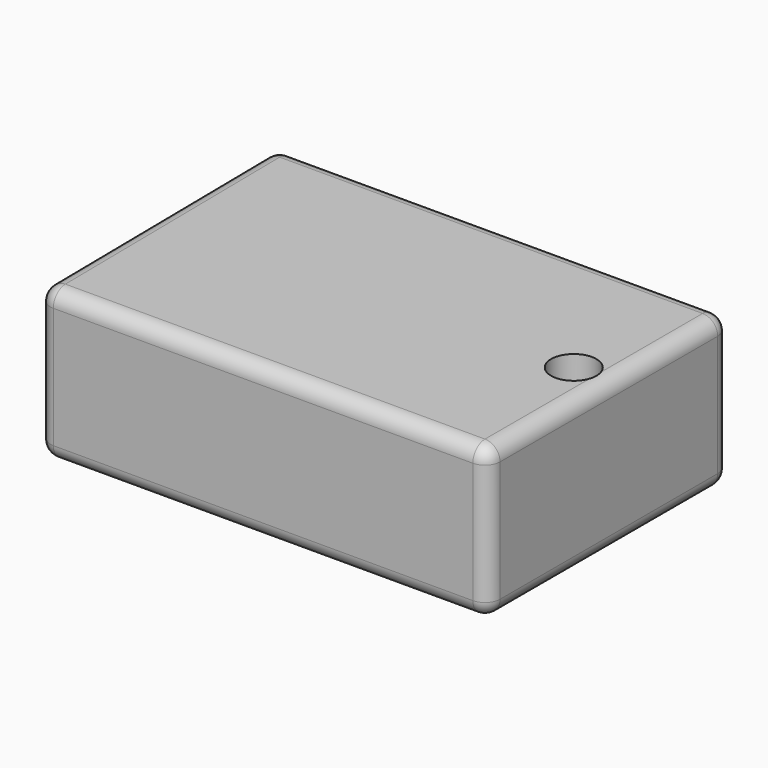
from build123d import *

# Parameters (mm, degrees)
F0_R         = 15
F1_DEPTH     = 100
F2_T1_DEPTH  = 180
F2_T3_DEPTH  = 277.5790250274
F2_T5_DEPTH  = 80
F2_T7_DEPTH  = 279.8718117474
F2_T9_DEPTH  = 180.014601827
F2_S13_W     = 10
F2_S13_H     = 10
F2_T14_DEPTH = 10
F2_S19_W     = 10
F2_S19_H     = 10
F2_T20_DEPTH = 10
F2_T26_DEPTH = 10
F2_S31_W     = 10
F2_S31_H     = 10
F2_T32_DEPTH = 10
F2_T38_DEPTH = 10
F2_S43_W     = 10
F2_S43_H     = 10
F2_T44_DEPTH = 10
F2_T50_DEPTH = 10
F2_T56_DEPTH = 10


# Not quite as in the source:
# - a fillet or chamfer that OpenCascade refuses, or shapes differently, is made with other operations: its cross-section is extruded or revolved along the edge and cut away or added


with BuildPart() as f1:
    # F0 (on Top) → F1 (new body)
    with BuildSketch(Plane.XY):
        Polygon((148.6140583592, 151.6970589757), (-151.3859416408, 151.6970589757), (-148.8384008408, -48.3029410243), (148.6140583592, -48.3029410243), align=None)
        with Locations((124.343521893, 52.9859960079)):
            Circle(F0_R, mode=Mode.SUBTRACT)
    extrude(amount=F1_DEPTH)

    # F2: fillet of radius 10 on 12 edges, made by hand

    # F2_s2 → F2_t1 (cut)
    with BuildSketch(Plane.XZ.offset(-141.6970589757)):
        with BuildLine():
            ThreePointArc((148.6140583592, 90), (145.6851261711, 97.0710678119), (138.6140583592, 100))
            Line((138.6140583592, 100), (148.6140583592, 100))
            Line((148.6140583592, 100), (148.6140583592, 90))
        make_face()
        with BuildLine():
            ThreePointArc((148.6140583592, 10), (145.6851261711, 2.9289321881), (138.6140583592, 0))
            Line((138.6140583592, 0), (148.6140583592, 0))
            Line((148.6140583592, 0), (148.6140583592, 10))
        make_face()
    extrude(amount=F2_T1_DEPTH, mode=Mode.SUBTRACT)

    # F2_s4 → F2_t3 (cut)
    with BuildSketch(Plane.YZ.offset(-138.9649666681)):
        with BuildLine():
            ThreePointArc((-48.3029410243, 90), (-45.3740088362, 97.0710678119), (-38.3029410243, 100))
            Line((-38.3029410243, 100), (-48.3029410243, 100))
            Line((-48.3029410243, 100), (-48.3029410243, 90))
        make_face()
        with BuildLine():
            ThreePointArc((-48.3029410243, 10), (-45.3740088362, 2.9289321881), (-38.3029410243, 0))
            Line((-38.3029410243, 0), (-48.3029410243, 0))
            Line((-48.3029410243, 0), (-48.3029410243, 10))
        make_face()
    extrude(amount=F2_T3_DEPTH, mode=Mode.SUBTRACT)

    # F2_s6 → F2_t5 (cut)
    with BuildSketch(Plane.XY.offset(10)):
        with BuildLine():
            ThreePointArc((138.6140583592, -48.3029410243), (145.6851261711, -45.3740088362), (148.6140583592, -38.3029410243))
            Line((148.6140583592, -38.3029410243), (148.6140583592, -48.3029410243))
            Line((148.6140583592, -48.3029410243), (138.6140583592, -48.3029410243))
        make_face()
        with BuildLine():
            ThreePointArc((148.6140583592, 141.6970589757), (145.6851261711, 148.7681267876), (138.6140583592, 151.6970589757))
            Line((138.6140583592, 151.6970589757), (148.6140583592, 151.6970589757))
            Line((148.6140583592, 151.6970589757), (148.6140583592, 141.6970589757))
        make_face()
        with BuildLine():
            ThreePointArc((-138.9649666681, -48.3029410243), (-145.9908592421, -45.4188972875), (-148.9641555213, -38.4303077322))
            Line((-148.9641555213, -38.4303077322), (-148.8384008408, -48.3029410243))
            Line((-148.8384008408, -48.3029410243), (-138.9649666681, -48.3029410243))
        make_face()
        with BuildLine():
            ThreePointArc((-141.2577533882, 151.6970589757), (-148.3737096513, 148.7229515496), (-151.2569422414, 141.5696922678))
            Line((-151.2569422414, 141.5696922678), (-151.3859416408, 151.6970589757))
            Line((-151.3859416408, 151.6970589757), (-141.2577533882, 151.6970589757))
        make_face()
    extrude(amount=F2_T5_DEPTH, mode=Mode.SUBTRACT)

    # F2_s8 → F2_t7 (cut)
    with BuildSketch(Plane.YZ.offset(-141.2577533882)):
        with BuildLine():
            ThreePointArc((151.6970589757, 10), (148.7681267876, 2.9289321881), (141.6970589757, 0))
            Line((141.6970589757, 0), (151.6970589757, 0))
            Line((151.6970589757, 0), (151.6970589757, 10))
        make_face()
        with BuildLine():
            ThreePointArc((151.6970589757, 90), (148.7681267876, 97.0710678119), (141.6970589757, 100))
            Line((141.6970589757, 100), (151.6970589757, 100))
            Line((151.6970589757, 100), (151.6970589757, 90))
        make_face()
    extrude(amount=F2_T7_DEPTH, mode=Mode.SUBTRACT)

    # F2_s10 → F2_t9 (cut)
    with BuildSketch(Plane(origin=(-1.8275176256, 143.4730800475, 0), x_dir=(0, 0, 1), z_dir=(0.0127366708, -0.9999188853, 0))):
        with BuildLine():
            ThreePointArc((10, 149.4415465191), (2.9289321881, 146.512614331), (0, 139.4415465191))
            Line((0, 139.4415465191), (0, 149.4415465191))
            Line((0, 149.4415465191), (10, 149.4415465191))
        make_face()
        with BuildLine():
            ThreePointArc((90, 149.4415465191), (97.0710678119, 146.512614331), (100, 139.4415465191))
            Line((100, 139.4415465191), (100, 149.4415465191))
            Line((100, 149.4415465191), (90, 149.4415465191))
        make_face()
    extrude(amount=F2_T9_DEPTH, mode=Mode.SUBTRACT)


with BuildPart() as f2_tool12:
    # F2_s13 → F2_t14 (new body)
    with BuildSketch(Plane.XZ.offset(38.3029410243)):
        with Locations((143.6140583592, 95)):
            Rectangle(F2_S13_W, F2_S13_H)
    extrude(amount=F2_T14_DEPTH)

    # F2_s15 → F2_t16 (revolve, cut)
    with BuildSketch(Plane(origin=(138.6140583592, -38.3029410243, 90), x_dir=(-0.7071067812, 0, -0.7071067812), z_dir=(-0.7071067812, 0, 0.7071067812))):
        with BuildLine():
            ThreePointArc((0, -10), (10, 0), (0, 10))
            Line((0, 10), (0, -10))
        make_face()
    revolve(axis=Axis((138.6140583592, -38.3029410243, 90), (0, -1, 0)), mode=Mode.SUBTRACT)


with BuildPart() as f1_1:
    add(f1.part)

    # F2_t11: cut F2_tool12
    add(f2_tool12.part, mode=Mode.SUBTRACT)


with BuildPart() as f2_tool18:
    # F2_s19 → F2_t20 (new body)
    with BuildSketch(Plane.YZ.offset(138.6140583592)):
        with Locations((146.6970589757, 95)):
            Rectangle(F2_S19_W, F2_S19_H)
    extrude(amount=F2_T20_DEPTH)

    # F2_s21 → F2_t22 (revolve, cut)
    with BuildSketch(Plane(origin=(138.6140583592, 141.6970589757, 90), x_dir=(0, -0.7071067812, -0.7071067812), z_dir=(0, -0.7071067812, 0.7071067812))):
        with BuildLine():
            ThreePointArc((0, -10), (10, 0), (0, 10))
            Line((0, 10), (0, -10))
        make_face()
    revolve(axis=Axis((138.6140583592, 141.6970589757, 90), (1, 0, 0)), mode=Mode.SUBTRACT)


with BuildPart() as f1_2:
    add(f1_1.part)

    # F2_t17: cut F2_tool18
    add(f2_tool18.part, mode=Mode.SUBTRACT)


with BuildPart() as f2_tool24:
    # F2_s25 → F2_t26 (new body)
    with BuildSketch(Plane.XY.offset(90)):
        Polygon((-138.9649666681, -38.3029410243), (-138.9649666681, -48.3029410243), (-148.8384008408, -48.3029410243), (-148.9641555213, -38.4303077322), align=None)
    extrude(amount=F2_T26_DEPTH)

    # F2_s27 → F2_t28 (revolve, cut)
    with BuildSketch(Plane(origin=(-138.9649666681, -38.3029410243, 90), x_dir=(0.7025892574, 0.7115956263, 0), z_dir=(0.7115956263, -0.7025892574, 0))):
        with BuildLine():
            ThreePointArc((0, -10), (10, 0), (0, 10))
            Line((0, 10), (0, -10))
        make_face()
    revolve(axis=Axis((-138.9649666681, -38.3029410243, 90), (0, 0, 1)), mode=Mode.SUBTRACT)


with BuildPart() as f1_3:
    add(f1_2.part)

    # F2_t23: cut F2_tool24
    add(f2_tool24.part, mode=Mode.SUBTRACT)


with BuildPart() as f2_tool30:
    # F2_s31 → F2_t32 (new body)
    with BuildSketch(Plane.XZ.offset(38.3029410243)):
        with Locations((143.6140583592, 5)):
            Rectangle(F2_S31_W, F2_S31_H)
    extrude(amount=F2_T32_DEPTH)

    # F2_s33 → F2_t34 (revolve, cut)
    with BuildSketch(Plane(origin=(138.6140583592, -38.3029410243, 10), x_dir=(-0.7071067812, 0, 0.7071067812), z_dir=(0.7071067812, 0, 0.7071067812))):
        with BuildLine():
            ThreePointArc((0, -10), (10, 0), (0, 10))
            Line((0, 10), (0, -10))
        make_face()
    revolve(axis=Axis((138.6140583592, -38.3029410243, 10), (0, -1, 0)), mode=Mode.SUBTRACT)


with BuildPart() as f1_4:
    add(f1_3.part)

    # F2_t29: cut F2_tool30
    add(f2_tool30.part, mode=Mode.SUBTRACT)


with BuildPart() as f2_tool36:
    # F2_s37 → F2_t38 (new body)
    with BuildSketch(Plane.XY.offset(10)):
        Polygon((-138.9649666681, -38.3029410243), (-138.9649666681, -48.3029410243), (-148.8384008408, -48.3029410243), (-148.9641555213, -38.4303077322), align=None)
    extrude(amount=-F2_T38_DEPTH)

    # F2_s39 → F2_t40 (revolve, cut)
    with BuildSketch(Plane(origin=(-138.9649666681, -38.3029410243, 10), x_dir=(0.7025892574, 0.7115956263, 0), z_dir=(-0.7115956263, 0.7025892574, 0))):
        with BuildLine():
            ThreePointArc((0, -10), (10, 0), (0, 10))
            Line((0, 10), (0, -10))
        make_face()
    revolve(axis=Axis((-138.9649666681, -38.3029410243, 10), (0, 0, -1)), mode=Mode.SUBTRACT)


with BuildPart() as f1_5:
    add(f1_4.part)

    # F2_t35: cut F2_tool36
    add(f2_tool36.part, mode=Mode.SUBTRACT)


with BuildPart() as f2_tool42:
    # F2_s43 → F2_t44 (new body)
    with BuildSketch(Plane.YZ.offset(138.6140583592)):
        with Locations((146.6970589757, 5)):
            Rectangle(F2_S43_W, F2_S43_H)
    extrude(amount=F2_T44_DEPTH)

    # F2_s45 → F2_t46 (revolve, cut)
    with BuildSketch(Plane(origin=(138.6140583592, 141.6970589757, 10), x_dir=(0, -0.7071067812, 0.7071067812), z_dir=(0, 0.7071067812, 0.7071067812))):
        with BuildLine():
            ThreePointArc((0, -10), (10, 0), (0, 10))
            Line((0, 10), (0, -10))
        make_face()
    revolve(axis=Axis((138.6140583592, 141.6970589757, 10), (1, 0, 0)), mode=Mode.SUBTRACT)


with BuildPart() as f1_6:
    add(f1_5.part)

    # F2_t41: cut F2_tool42
    add(f2_tool42.part, mode=Mode.SUBTRACT)


with BuildPart() as f2_tool48:
    # F2_s49 → F2_t50 (new body)
    with BuildSketch(Plane.XY.offset(10)):
        Polygon((-141.2577533882, 141.6970589757), (-141.2577533882, 151.6970589757), (-151.3859416408, 151.6970589757), (-151.2569422414, 141.5696922678), align=None)
    extrude(amount=-F2_T50_DEPTH)

    # F2_s51 → F2_t52 (revolve, cut)
    with BuildSketch(Plane(origin=(-141.2577533882, 141.6970589757, 10), x_dir=(0.7115956263, -0.7025892574, 0), z_dir=(0.7025892574, 0.7115956263, 0))):
        with BuildLine():
            ThreePointArc((0, -10), (10, 0), (0, 10))
            Line((0, 10), (0, -10))
        make_face()
    revolve(axis=Axis((-141.2577533882, 141.6970589757, 10), (0, 0, -1)), mode=Mode.SUBTRACT)


with BuildPart() as f1_7:
    add(f1_6.part)

    # F2_t47: cut F2_tool48
    add(f2_tool48.part, mode=Mode.SUBTRACT)


with BuildPart() as f2_tool54:
    # F2_s55 → F2_t56 (new body)
    with BuildSketch(Plane.XY.offset(90)):
        Polygon((-141.2577533882, 141.6970589757), (-141.2577533882, 151.6970589757), (-151.3859416408, 151.6970589757), (-151.2569422414, 141.5696922678), align=None)
    extrude(amount=F2_T56_DEPTH)

    # F2_s57 → F2_t58 (revolve, cut)
    with BuildSketch(Plane(origin=(-141.2577533882, 141.6970589757, 90), x_dir=(0.7115956263, -0.7025892574, 0), z_dir=(-0.7025892574, -0.7115956263, 0))):
        with BuildLine():
            ThreePointArc((0, -10), (10, 0), (0, 10))
            Line((0, 10), (0, -10))
        make_face()
    revolve(axis=Axis((-141.2577533882, 141.6970589757, 90), (0, 0, 1)), mode=Mode.SUBTRACT)


with BuildPart() as f1_8:
    add(f1_7.part)

    # F2_t53: cut F2_tool54
    add(f2_tool54.part, mode=Mode.SUBTRACT)


solid = f1_8.part
